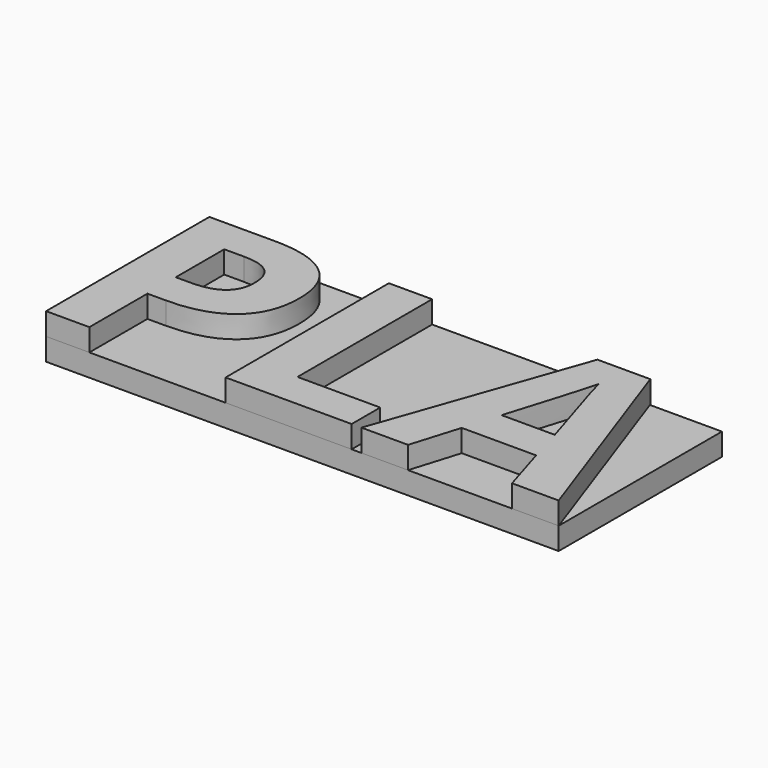
from build123d import *

# Parameters (mm, degrees)
F0_TEXT_SIZE = 25.6698219156
F1_DEPTH     = 2
F3_DEPTH     = 2


# Not quite as in the source:
# - Text() gives the source's letters only with a copy of the font that has no kerning and outlines rounded to 1/6400 em; it was checked with that copy


with BuildPart() as f1:
    # F0 (on Top) → F1 (new body)
    with BuildSketch(Plane.XY):
        with Locations((-25, 0)):
            Text('PLA', F0_TEXT_SIZE, font='Open Sans', font_style=FontStyle.BOLD, text_align=(TextAlign.LEFT, TextAlign.BOTTOM))
    extrude(amount=F1_DEPTH)


with BuildPart() as f3:
    # F2 (on Top) → F3 (new body)
    with BuildSketch(Plane.XY):
        with BuildLine():
            add(Edge.make_bspline(
                [(-13.5047328734, 18.3258463019), (-12.5331817539, 17.8971700019), (-11.7700144393, 16.8899406385)],
                knots=[3.337076849, 3.337076849, 3.337076849, 5.5889811809, 5.5889811809, 5.5889811809], degree=2))
            add(Edge.make_bspline(
                [(-11.7700144393, 16.8899406385), (-8.9399831658, 15.6733466868), (-10.0352960051, 12.610300016)],
                knots=[0, 0, 0, 5.095639291, 5.095639291, 5.095639291], degree=2))
            add(Edge.make_bspline(
                [(-10.0352960051, 12.610300016), (-8.9059759301, 9.3952447991), (-11.884325365, 8.0839884486)],
                knots=[0, 0, 0, 5.3832889827, 5.3832889827, 5.3832889827], degree=2))
            add(Edge.make_bspline(
                [(-11.884325365, 8.0839884486), (-13.8224433068, 5.4159359408), (-17.142627948, 6.5177282208)],
                knots=[0, 0, 0, 5.8325108663, 5.8325108663, 5.8325108663], degree=2))
            Line((-17.142627948, 6.5177282208), (-18.8071554629, 6.5177282208))
            Line((-18.8071554629, 6.5177282208), (-18.8071554629, 0))
            Line((-18.8071554629, 0), (-6.5738809562, 0))
            Line((-6.5738809562, 0), (-6.5738809562, 18.3258463019))
            Line((-6.5738809562, 18.3258463019), (-13.5047328734, 18.3258463019))
        make_face()
        with BuildLine():
            add(Edge.make_bspline(
                [(-11.7700144393, 16.8899406385), (-8.9399831658, 15.6733466868), (-10.0352960051, 12.610300016)],
                knots=[0, 0, 0, 5.095639291, 5.095639291, 5.095639291], degree=2))
            add(Edge.make_bspline(
                [(-13.5047328734, 18.3258463019), (-12.5331817539, 17.8971700019), (-11.7700144393, 16.8899406385)],
                knots=[3.337076849, 3.337076849, 3.337076849, 5.5889811809, 5.5889811809, 5.5889811809], degree=2))
            Line((-13.5047328734, 18.3258463019), (-16.8418097224, 18.3258463019))
            Line((-16.8418097224, 18.3258463019), (-22.6937269373, 18.3258463019))
            Line((-22.6937269373, 18.3258463019), (-22.6937269373, 0))
            Line((-22.6937269373, 0), (-18.8071554629, 0))
            Line((-18.8071554629, 0), (-18.8071554629, 6.5177282208))
            Line((-18.8071554629, 6.5177282208), (-17.142627948, 6.5177282208))
            add(Edge.make_bspline(
                [(-11.884325365, 8.0839884486), (-13.8224433068, 5.4159359408), (-17.142627948, 6.5177282208)],
                knots=[0, 0, 0, 5.8325108663, 5.8325108663, 5.8325108663], degree=2))
            add(Edge.make_bspline(
                [(-10.0352960051, 12.610300016), (-8.9059759301, 9.3952447991), (-11.884325365, 8.0839884486)],
                knots=[0, 0, 0, 5.3832889827, 5.3832889827, 5.3832889827], degree=2))
        make_face()
        Polygon((-2.6873094818, 18.3258463019), (-6.5738809562, 18.3258463019), (-6.5738809562, 0), (4.7449061447, 0), (4.7449061447, 3.2087277395), (-2.6873094818, 3.2087277395), align=None)
        Polygon((12.0661005258, 18.3258463019), (-2.6873094818, 18.3258463019), (-2.6873094818, 3.2087277395), (4.7449061447, 3.2087277395), (4.7449061447, 0), (5.6232953634, 0), align=None)
        Polygon((16.8687015255, 18.3258463019), (12.0661005258, 18.3258463019), (5.6232953634, 0), (9.8106850634, 0), (11.1382961656, 4.3638697257), (17.820471683, 4.3638697257), (19.1480827852, 0), (23.3354724852, 0), align=None)
        Polygon((12.0928926681, 18.4020535858), (12.0661005258, 18.3258463019), (16.8687015255, 18.3258463019), (16.8418097224, 18.4020535858), align=None)
        Polygon((23.3354724852, 18.3258463019), (16.8687015255, 18.3258463019), (23.3354724852, 0), align=None)
        Polygon((11.1382961656, 4.3638697257), (9.8106850634, 0), (19.1480827852, 0), (17.820471683, 4.3638697257), align=None)
    extrude(amount=-F3_DEPTH)


solid = Compound([f1.part, f3.part])
